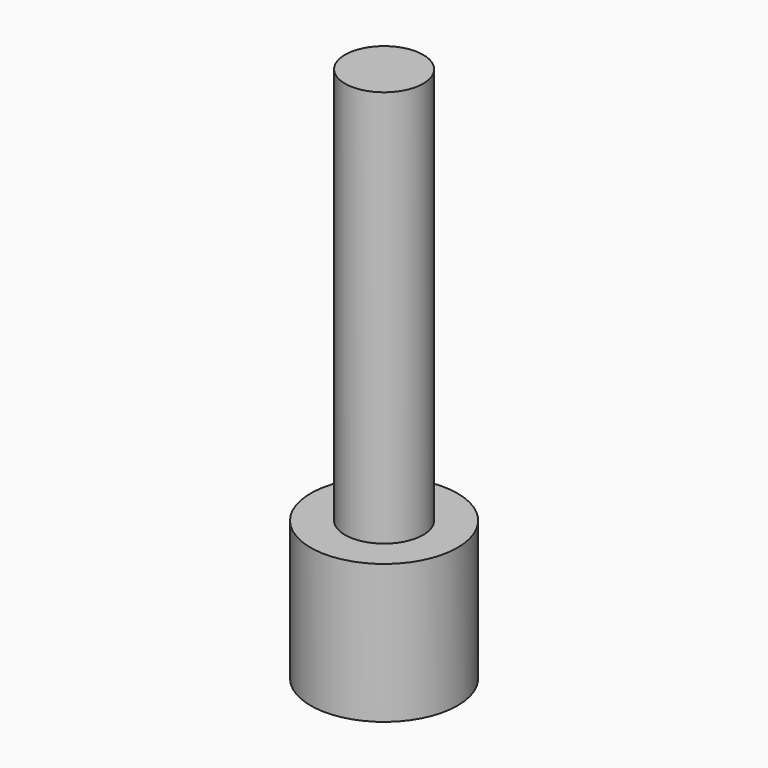
from build123d import *

# Parameters (mm, degrees)
F0_R     = 4.699
F1_DEPTH = 8.89
F2_R     = 2.5
F3_DEPTH = 25.4
F4_R     = 3.556
F5_DEPTH = 6.35


# Not quite as in the source:
# - a feature names something its author has since deleted; it is built from what else it names


with BuildPart() as f1:
    # F0 (on Top) → F1 (new body)
    with BuildSketch(Plane.XY):
        Circle(F0_R)
    extrude(amount=F1_DEPTH)

    # F2 (on face) → F3 (join)
    with BuildSketch(Plane.XY.offset(8.89)):
        Circle(F2_R)
    extrude(amount=F3_DEPTH)

    # F4 (on face) → F5 (cut)
    with BuildSketch(Plane(origin=(0, 0, 0), x_dir=(1, 0, 0), z_dir=(0, 0, -1))):
        Circle(F4_R)
    extrude(amount=-F5_DEPTH, mode=Mode.SUBTRACT)


solid = f1.part
